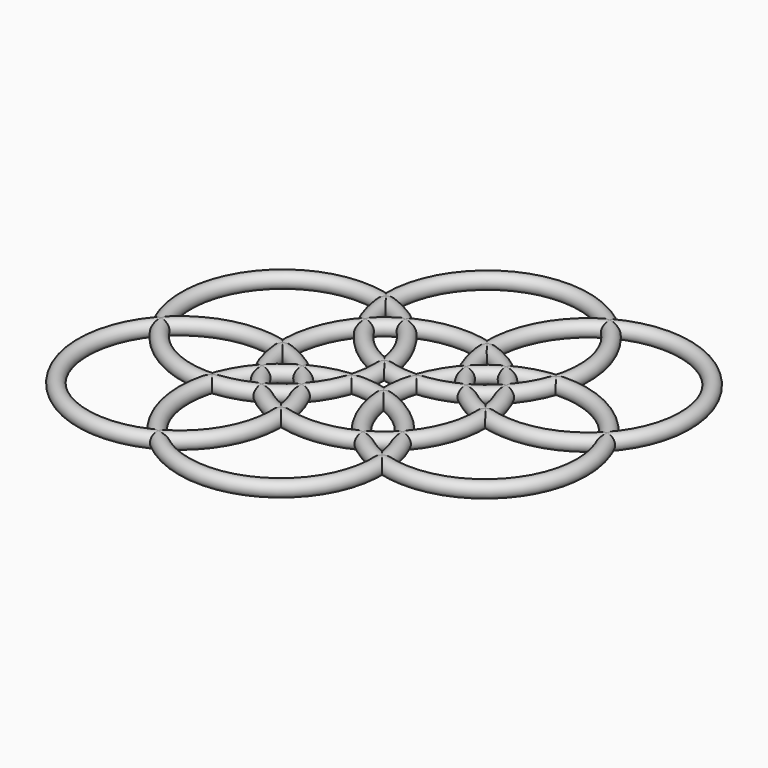
from build123d import *

# Parameters (mm, degrees)
F1_R             = 7.2773977025
F2_COPIES_COUNT  = 4
F2_COPIES1_COUNT = 4


# Not quite as in the source:
# - a pattern or mirror of a feature is missing from the dataset's text; its kind, count and spacing are read off the source's solid


with BuildPart() as f2:
    # F1 (on Right) → F2 (revolve)
    with BuildSketch(Plane.YZ):
        with Locations((-92.4350097775, 0)):
            Circle(F1_R)
    revolve(axis=Axis((0, 0, 0), (0, 0, 1)))


with BuildPart() as f2_copies_1:
    # F2_copies: instance of F2
    add(f2.part.rotate(Axis((60.011318, 46.958298, 0), (0, 0, 1)), 1 * 360 / F2_COPIES_COUNT))


with BuildPart() as f2_copies_2:
    # F2_copies: instance of F2
    add(f2.part.rotate(Axis((60.011318, 46.958298, 0), (0, 0, 1)), 2 * 360 / F2_COPIES_COUNT))


with BuildPart() as f2_copies_3:
    # F2_copies: instance of F2
    add(f2.part.rotate(Axis((60.011318, 46.958298, 0), (0, 0, 1)), 3 * 360 / F2_COPIES_COUNT))


with BuildPart() as f2_copies1_1:
    # F2_copies1: instance of F2
    add(f2.part.rotate(Axis((-60.011318, -46.958298, 0), (0, 0, 1)), 1 * 360 / F2_COPIES1_COUNT))


with BuildPart() as f2_copies1_2:
    # F2_copies1: instance of F2
    add(f2.part.rotate(Axis((-60.011318, -46.958298, 0), (0, 0, 1)), 2 * 360 / F2_COPIES1_COUNT))


with BuildPart() as f2_copies1_3:
    # F2_copies1: instance of F2
    add(f2.part.rotate(Axis((-60.011318, -46.958298, 0), (0, 0, 1)), 3 * 360 / F2_COPIES1_COUNT))


solid = Compound([f2.part, f2_copies_1.part, f2_copies_2.part, f2_copies_3.part, f2_copies1_1.part, f2_copies1_2.part, f2_copies1_3.part])
